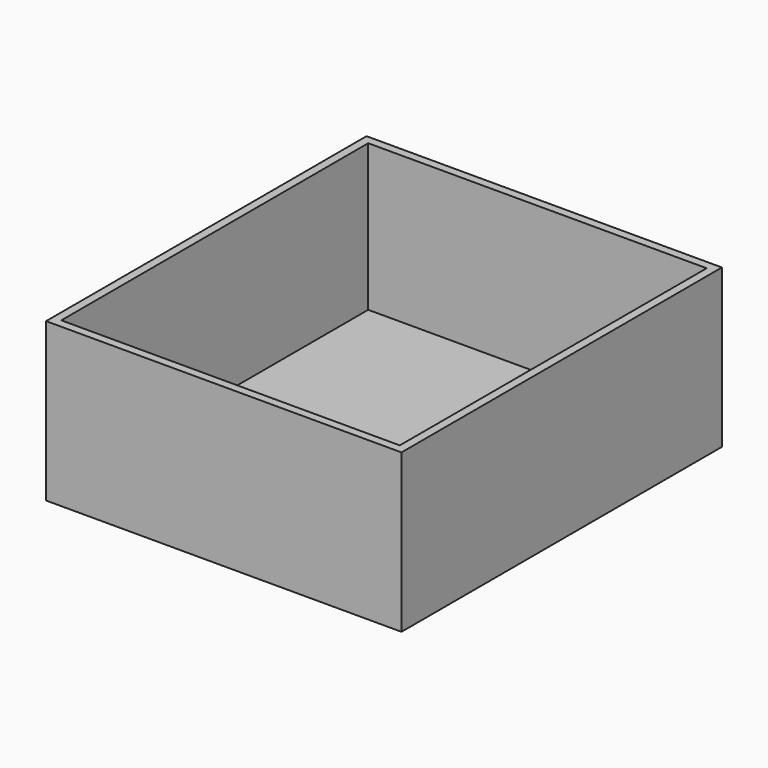
from build123d import *

# Parameters (mm, degrees)
F0_W     = 63
F0_H     = 71
F0_W_2   = 60
F0_H_2   = 68
F0_R     = 1.5
F1_DEPTH = 2
F2_DEPTH = 28


with BuildPart() as f1:
    # F0 (on Top) → F1 (new body)
    with BuildSketch(Plane.XY):
        Rectangle(F0_W, F0_H)
        Rectangle(F0_W_2, F0_H_2, mode=Mode.SUBTRACT)
        Rectangle(F0_W_2, F0_H_2)
        Circle(F0_R, mode=Mode.SUBTRACT)
    extrude(amount=F1_DEPTH)

    # F0 (on Top) → F2 (join)
    with BuildSketch(Plane.XY):
        Rectangle(F0_W, F0_H)
        Rectangle(F0_W_2, F0_H_2, mode=Mode.SUBTRACT)
    extrude(amount=F2_DEPTH)


solid = f1.part
